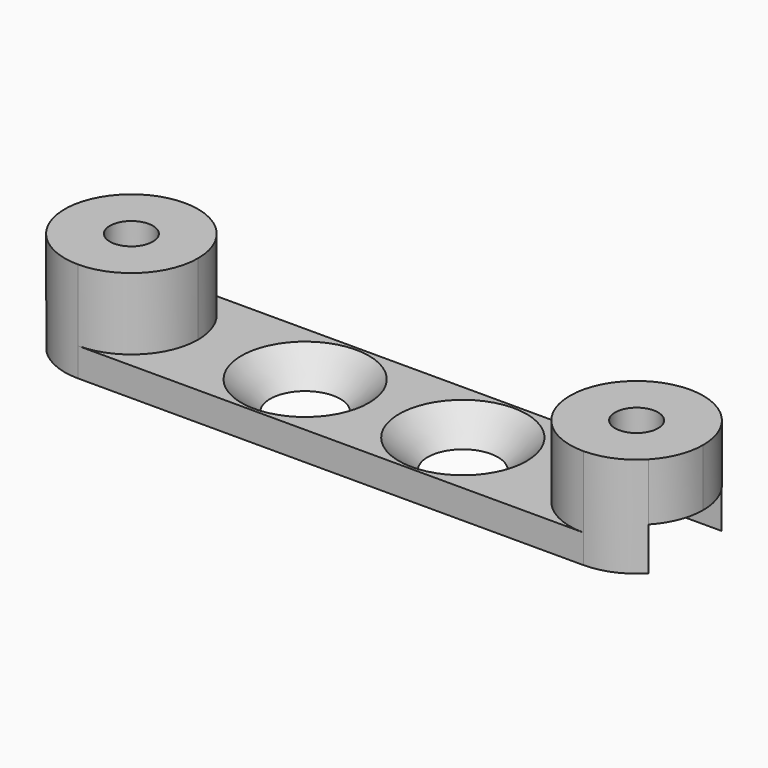
from build123d import *

# Parameters (mm, degrees)
F0_R     = 1.5
F1_DEPTH = 7
F0_R_2   = 2.15
F2_DEPTH = 2
F4_DEPTH = 3


# Not quite as in the source:
# - a fillet or chamfer that OpenCascade refuses, or shapes differently, is made with other operations: its cross-section is extruded or revolved along the edge and cut away or added
# - ends of sketch curves that miss each other by under 0.0002 mm in the source are joined
# - a feature names something its author has since deleted; it is built from what else it names


with BuildPart() as f1:
    # F0 (on Top) → F1 (new body)
    with BuildSketch(Plane.XY):
        with BuildLine():
            Line((-15.7774791386, 3.2), (-20.9987960816, 3.2))
            ThreePointArc((-20.9987960816, 3.2), (-22.275, 0), (-20.9987960816, -3.2))
            Line((-20.9987960816, -3.2), (-15.7774791386, -3.2))
            Line((-15.7774791386, -3.2), (-13.9299582772, 0))
            Line((-13.9299582772, 0), (-15.7774791386, 3.2))
        make_face()
        with Locations((-17.625, 0)):
            Circle(F0_R, mode=Mode.SUBTRACT)
        with BuildLine():
            ThreePointArc((-17.625, -4.65), (-14.3369534675, -3.2880465325), (-12.975, 0))
            ThreePointArc((-12.975, 0), (-14.3369534675, 3.2880465325), (-17.625, 4.65))
            ThreePointArc((-17.625, 4.65), (-19.4610964027, 4.2721481716), (-20.9987960816, 3.2))
            Line((-20.9987960816, 3.2), (-15.7774791386, 3.2))
            Line((-15.7774791386, 3.2), (-13.9299582772, 0))
            Line((-13.9299582772, 0), (-15.7774791386, -3.2))
            Line((-15.7774791386, -3.2), (-20.9987960816, -3.2))
            ThreePointArc((-20.9987960816, -3.2), (-19.4610964027, -4.2721481716), (-17.625, -4.65))
        make_face()
    extrude(amount=F1_DEPTH)


with BuildPart() as f1b:
    # F0 (on Top) → F1, piece 2 (new body)
    with BuildSketch(Plane.XY):
        with BuildLine():
            ThreePointArc((20.9987962368, 3.1999998363), (19.4610965063, 4.272148127), (17.625, 4.65))
            ThreePointArc((17.625, 4.65), (12.975, 0), (17.625, -4.65))
            ThreePointArc((17.625, -4.65), (19.4610965063, -4.272148127), (20.9987962368, -3.1999998363))
            Line((20.9987962368, -3.1999998363), (15.7774794664, -3.2))
            Line((15.7774794664, -3.2), (13.929958605, 0))
            Line((13.929958605, 0), (15.7774794664, 3.2))
            Line((15.7774794664, 3.2), (20.9987962368, 3.1999998363))
        make_face()
        with BuildLine():
            ThreePointArc((22.275, 0), (21.9441812014, 1.7225486203), (20.9987962368, 3.1999998363))
            Line((20.9987962368, 3.1999998363), (15.7774794664, 3.2))
            Line((15.7774794664, 3.2), (13.929958605, 0))
            Line((13.929958605, 0), (15.7774794664, -3.2))
            Line((15.7774794664, -3.2), (20.9987964094, -3.2))
            ThreePointArc((20.9987964094, -3.2), (21.9441812014, -1.7225486203), (22.275, 0))
        make_face()
        with Locations((17.625, 0)):
            Circle(F0_R, mode=Mode.SUBTRACT)
    extrude(amount=F1_DEPTH)


with BuildPart() as f2:
    # F0 (on Top) → F2 (new body)
    with BuildSketch(Plane.XY):
        with BuildLine():
            ThreePointArc((-17.625, 4.65), (-14.3369534675, 3.2880465325), (-12.975, 0))
            ThreePointArc((-12.975, 0), (-14.3369534675, -3.2880465325), (-17.625, -4.65))
            Line((-17.625, -4.65), (17.625, -4.65))
            ThreePointArc((17.625, -4.65), (12.975, 0), (17.625, 4.65))
            Line((17.625, 4.65), (-17.625, 4.65))
        make_face()
        with Locations((-5.5, 0)):
            Circle(F0_R_2, mode=Mode.SUBTRACT)
        with Locations((5.5, 0)):
            Circle(F0_R_2, mode=Mode.SUBTRACT)
    extrude(amount=F2_DEPTH)

    # F3: chamfer of 2.3 on 2 edges, made by hand

    # F3_s1 → F3_t2 (revolve, cut)
    with BuildSketch(Plane.XZ):
        Polygon((-3.35, -0.3), (-1.05, 2), (-3.35, 2), align=None)
    revolve(axis=Axis((-5.5, 0, 2), (0, 0, 1)), mode=Mode.SUBTRACT)

    # F3_s3 → F3_t4 (revolve, cut)
    with BuildSketch(Plane.XZ):
        Polygon((7.65, -0.3), (9.95, 2), (7.65, 2), align=None)
    revolve(axis=Axis((5.5, 0, 2), (0, 0, 1)), mode=Mode.SUBTRACT)


with BuildPart() as f4_tool:
    # F0 (on Top) → F4 (new body)
    with BuildSketch(Plane.XY):
        with BuildLine():
            Line((-15.7774791386, 3.2), (-20.9987960816, 3.2))
            ThreePointArc((-20.9987960816, 3.2), (-22.275, 0), (-20.9987960816, -3.2))
            Line((-20.9987960816, -3.2), (-15.7774791386, -3.2))
            Line((-15.7774791386, -3.2), (-13.9299582772, 0))
            Line((-13.9299582772, 0), (-15.7774791386, 3.2))
        make_face()
        with Locations((-17.625, 0)):
            Circle(F0_R, mode=Mode.SUBTRACT)
        with BuildLine():
            ThreePointArc((22.275, 0), (21.9441812014, 1.7225486203), (20.9987962368, 3.1999998363))
            Line((20.9987962368, 3.1999998363), (15.7774794664, 3.2))
            Line((15.7774794664, 3.2), (13.929958605, 0))
            Line((13.929958605, 0), (15.7774794664, -3.2))
            Line((15.7774794664, -3.2), (20.9987964094, -3.2))
            ThreePointArc((20.9987964094, -3.2), (21.9441812014, -1.7225486203), (22.275, 0))
        make_face()
        with Locations((17.625, 0)):
            Circle(F0_R, mode=Mode.SUBTRACT)
    extrude(amount=F4_DEPTH)


with BuildPart() as f1_1:
    add(f1.part)

    # F4: cut by f4_tool
    add(f4_tool.part, mode=Mode.SUBTRACT)


with BuildPart() as f1b_1:
    add(f1b.part)

    # F4: cut by f4_tool
    add(f4_tool.part, mode=Mode.SUBTRACT)


solid = Compound([f2.part, f1_1.part, f1b_1.part])
